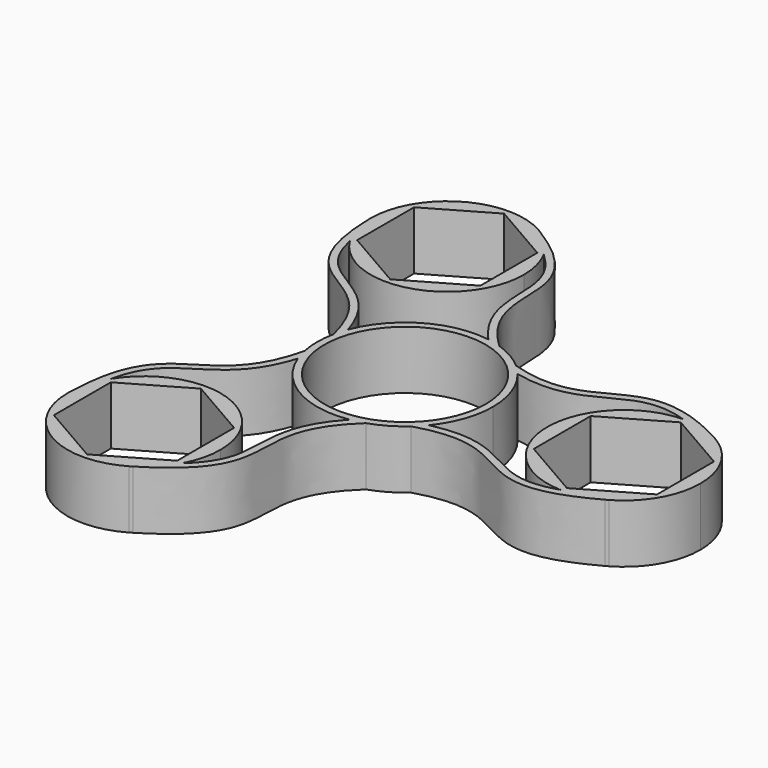
from build123d import *

# Parameters (mm, degrees)
F1_R     = 11.05
F2_DEPTH = 8


# Not quite as in the source:
# - the dataset's text gives a spline's control points without its knots; the knots are read off the source's solid


with BuildPart() as f2:
    # F1 (on Top) → F2 (new body)
    with BuildSketch(Plane.XY):
        with BuildLine():
            add(Edge.make_bspline(
                [(-23.9498664284, -20.4898704816), (-23.8093874058, -19.8426867285), (-23.468726692, -18.6366109287), (-22.828701594, -17.1870085553), (-22.0677112404, -16.020381617), (-21.2122966171, -15.0814244691), (-20.2601756399, -14.2881589816), (-18.8658523772, -13.3343486428), (-16.9218620299, -12.1842349069), (-14.8947876528, -10.62274426), (-13.3989040624, -8.8483289097), (-12.2627989857, -7.0040651939), (-11.5948300671, -5.3682178456), (-11.2616482193, -4.2869312315)],
                knots=[0.1298047456, 0.1298047456, 0.1298047456, 0.1298047456, 0.1875, 0.25, 0.3125, 0.375, 0.4375, 0.5, 0.625, 0.75, 0.8125, 0.875, 0.9599937126, 0.9599937126, 0.9599937126, 0.9599937126], degree=3))
            ThreePointArc((-11.2616482193, -4.2869312315), (-11.5680523877, -3.3738203797), (-11.8005517613, -2.4391552079))
            add(Edge.make_bspline(
                [(-25.4913456153, -25.5545377836), (-25.0594663371, -8.3982224046), (-14.9740294657, -16.111652051), (-11.8005517613, -2.4391552079)],
                knots=[0.221092115, 0.221092115, 0.221092115, 0.221092115, 27.237513428, 27.237513428, 27.237513428, 27.237513428], degree=3))
            ThreePointArc((-25.4913456153, -25.5545377836), (-25.0450433126, -22.923458588), (-23.9498664284, -20.4898704816))
        make_face()
        with BuildLine():
            add(Edge.make_bspline(
                [(3.7879055068, -11.4391552079), (-6.4660852403, -21.0237159398), (5.2566592195, -25.9012456555), (-9.3852060949, -34.8534217713)],
                knots=[0, 0, 0, 0, 27.016421313, 27.016421313, 27.016421313, 27.016421313], degree=3))
            ThreePointArc((3.7879055068, -11.4391552079), (2.8622120372, -11.70513743), (1.9182327589, -11.8963390622))
            add(Edge.make_bspline(
                [(1.9182327589, -11.8963390622), (1.1484020062, -12.7255263135), (0.0657011052, -14.12192804), (-0.9634255856, -16.0279557557), (-1.7521725606, -18.2106366213), (-2.0909259401, -20.7468798507), (-2.114958479, -23.0054817441), (-2.2438208314, -24.6899062801), (-2.454748407, -25.9110999776), (-2.8402018384, -27.1213893461), (-3.4700352269, -28.3637397934), (-4.4054151587, -29.6428189741), (-5.2795770833, -30.5408777063), (-5.7698151431, -30.9861279851)],
                knots=[0.0400062874, 0.0400062874, 0.0400062874, 0.0400062874, 0.125, 0.1875, 0.25, 0.375, 0.5, 0.5625, 0.625, 0.6875, 0.75, 0.8125, 0.8701952544, 0.8701952544, 0.8701952544, 0.8701952544], degree=3))
            ThreePointArc((-5.7698151431, -30.9861279851), (-7.3297758235, -33.1513730416), (-9.3852060949, -34.8534217713))
        make_face()
        with BuildLine():
            ThreePointArc((9.3434154605, 7.6094078307), (8.7058403505, 8.3313170502), (8.0126462545, 9))
            ThreePointArc((8.0126462545, 9), (6.025, 10.4356061156), (3.7879055068, 11.4391552079))
            ThreePointArc((3.7879055068, 11.4391552079), (2.8622120372, 11.70513743), (1.9182327589, 11.8963390622))
            ThreePointArc((1.9182327589, 11.8963390622), (-6.025, 10.4356061156), (-11.2616482193, 4.2869312315))
            ThreePointArc((-11.2616482193, 4.2869312315), (-11.5680523877, 3.3738203797), (-11.8005517613, 2.4391552079))
            ThreePointArc((-11.8005517613, 2.4391552079), (-12.05, 0), (-11.8005517613, -2.4391552079))
            ThreePointArc((-11.8005517613, -2.4391552079), (-11.5680523877, -3.3738203797), (-11.2616482193, -4.2869312315))
            ThreePointArc((-11.2616482193, -4.2869312315), (-6.025, -10.4356061156), (1.9182327589, -11.8963390622))
            ThreePointArc((1.9182327589, -11.8963390622), (2.8622120372, -11.70513743), (3.7879055068, -11.4391552079))
            ThreePointArc((3.7879055068, -11.4391552079), (6.025, -10.4356061156), (8.0126462545, -9))
            ThreePointArc((8.0126462545, -9), (8.7058403505, -8.3313170502), (9.3434154605, -7.6094078307))
            ThreePointArc((9.3434154605, -7.6094078307), (11.3532078352, -4.0382139432), (12.05, 0))
            ThreePointArc((12.05, 0), (11.3532078352, 4.0382139432), (9.3434154605, 7.6094078307))
        make_face()
        Circle(F1_R, mode=Mode.SUBTRACT)
        with BuildLine():
            add(Edge.make_bspline(
                [(-9.3852060949, -34.8534217713), (-9.5050295509, -34.9266829753), (-9.6266186878, -35.0002170649), (-9.75, -35.0740288533)],
                knots=[27.016421313, 27.016421313, 27.016421313, 27.016421313, 27.237513428, 27.237513428, 27.237513428, 27.237513428], degree=3))
            ThreePointArc((-9.3852060949, -34.8534217713), (-7.3297758235, -33.1513730416), (-5.7698151431, -30.9861279851))
            ThreePointArc((-5.7698151431, -30.9861279851), (-4.8224035009, -28.5627244489), (-4.5, -25.9807621135))
            ThreePointArc((-4.5, -25.9807621135), (-12.1472467245, -15.8757238281), (-23.9498664284, -20.4898704816))
            ThreePointArc((-23.9498664284, -20.4898704816), (-25.0450433126, -22.923458588), (-25.4913456153, -25.5545377836))
            add(Edge.make_bspline(
                [(-25.5, -25.9807621135), (-25.4977677723, -25.8370048686), (-25.4948799511, -25.6949385424), (-25.4913456153, -25.5545377836)],
                knots=[0, 0, 0, 0, 0.221092115, 0.221092115, 0.221092115, 0.221092115], degree=3))
            ThreePointArc((-25.5, -25.9807621135), (-20.25, -35.0740288533), (-9.75, -35.0740288533))
        make_face()
        Polygon((-23.45, -21.1021523389), (-15, -16.2235425642), (-6.55, -21.1021523389), (-6.55, -30.8593718882), (-15, -35.7379816628), (-23.45, -30.8593718882), align=None, mode=Mode.SUBTRACT)
        with BuildLine():
            ThreePointArc((35.25, -9.0932667397), (39.0932667397, -5.25), (40.5, 0))
            ThreePointArc((40.5, 0), (39.0932667397, 5.25), (35.25, 9.0932667397))
            add(Edge.make_bspline(
                [(34.8765517102, 9.2988839877), (34.9999095019, 9.2317444329), (35.1243864601, 9.1632121963), (35.25, 9.0932667397)],
                knots=[27.016421313, 27.016421313, 27.016421313, 27.016421313, 27.237513428, 27.237513428, 27.237513428, 27.237513428], degree=3))
            ThreePointArc((34.8765517102, 9.2988839877), (32.3748191361, 10.2279144536), (29.7196815716, 10.4962575034))
            ThreePointArc((29.7196815716, 10.4962575034), (19.5, 0), (29.7196815716, -10.4962575034))
            ThreePointArc((29.7196815716, -10.4962575034), (32.3748191361, -10.2279144536), (34.8765517102, -9.2988839877))
            add(Edge.make_bspline(
                [(34.8765517102, -9.2988839877), (34.9999095019, -9.2317444329), (35.1243864601, -9.1632121963), (35.25, -9.0932667397)],
                knots=[27.016421313, 27.016421313, 27.016421313, 27.016421313, 27.237513428, 27.237513428, 27.237513428, 27.237513428], degree=3))
        make_face()
        Polygon((21.55, 4.8786097747), (30, 9.7572195493), (38.45, 4.8786097747), (38.45, -4.8786097747), (30, -9.7572195493), (21.55, -4.8786097747), align=None, mode=Mode.SUBTRACT)
        with BuildLine():
            add(Edge.make_bspline(
                [(8.0126462545, -9), (21.440114706, -4.9120638887), (19.8028071176, -17.5030232509), (34.8765517102, -9.2988839877)],
                knots=[0, 0, 0, 0, 27.016421313, 27.016421313, 27.016421313, 27.016421313], degree=3))
            ThreePointArc((34.8765517102, -9.2988839877), (32.3748191361, -10.2279144536), (29.7196815716, -10.4962575034))
            add(Edge.make_bspline(
                [(9.3434154605, -7.6094078307), (10.4464280609, -7.3573084679), (12.1970978805, -7.1178628462), (14.362329648, -7.1796268461), (16.6469602135, -7.5878923613), (19.01278797, -8.5626449438), (20.9808108562, -9.6711331013), (22.5039964713, -10.4017472985), (23.6670450241, -10.8296755084), (24.9079130788, -11.1010077291), (26.2987368209, -11.1767312382), (27.8741418507, -11.0062080454), (29.0889644891, -10.6981909778), (29.7196815716, -10.4962575034)],
                knots=[0.0400062874, 0.0400062874, 0.0400062874, 0.0400062874, 0.125, 0.1875, 0.25, 0.375, 0.5, 0.5625, 0.625, 0.6875, 0.75, 0.8125, 0.8701952544, 0.8701952544, 0.8701952544, 0.8701952544], degree=3))
            ThreePointArc((9.3434154605, -7.6094078307), (8.7058403505, -8.3313170502), (8.0126462545, -9))
        make_face()
        with BuildLine():
            ThreePointArc((29.7196815716, 10.4962575034), (32.3748191361, 10.2279144536), (34.8765517102, 9.2988839877))
            add(Edge.make_bspline(
                [(8.0126462545, 9), (21.440114706, 4.9120638887), (19.8028071176, 17.5030232509), (34.8765517102, 9.2988839877)],
                knots=[0, 0, 0, 0, 27.016421313, 27.016421313, 27.016421313, 27.016421313], degree=3))
            ThreePointArc((8.0126462545, 9), (8.7058403505, 8.3313170502), (9.3434154605, 7.6094078307))
            add(Edge.make_bspline(
                [(9.3434154605, 7.6094078307), (10.4464280609, 7.3573084679), (12.1970978805, 7.1178628462), (14.362329648, 7.1796268461), (16.6469602135, 7.5878923613), (19.01278797, 8.5626449438), (20.9808108562, 9.6711331013), (22.5039964713, 10.4017472985), (23.6670450241, 10.8296755084), (24.9079130788, 11.1010077291), (26.2987368209, 11.1767312382), (27.8741418507, 11.0062080454), (29.0889644891, 10.6981909778), (29.7196815716, 10.4962575034)],
                knots=[0.0400062874, 0.0400062874, 0.0400062874, 0.0400062874, 0.125, 0.1875, 0.25, 0.375, 0.5, 0.5625, 0.625, 0.6875, 0.75, 0.8125, 0.8701952544, 0.8701952544, 0.8701952544, 0.8701952544], degree=3))
        make_face()
        with BuildLine():
            ThreePointArc((-11.8005517613, 2.4391552079), (-11.5680523877, 3.3738203797), (-11.2616482193, 4.2869312315))
            add(Edge.make_bspline(
                [(-23.9498664284, 20.4898704816), (-23.8093874058, 19.8426867285), (-23.468726692, 18.6366109287), (-22.828701594, 17.1870085553), (-22.0677112404, 16.020381617), (-21.2122966171, 15.0814244691), (-20.2601756399, 14.2881589816), (-18.8658523772, 13.3343486428), (-16.9218620299, 12.1842349069), (-14.8947876528, 10.62274426), (-13.3989040624, 8.8483289097), (-12.2627989857, 7.0040651939), (-11.5948300671, 5.3682178456), (-11.2616482193, 4.2869312315)],
                knots=[0.1298047456, 0.1298047456, 0.1298047456, 0.1298047456, 0.1875, 0.25, 0.3125, 0.375, 0.4375, 0.5, 0.625, 0.75, 0.8125, 0.875, 0.9599937126, 0.9599937126, 0.9599937126, 0.9599937126], degree=3))
            ThreePointArc((-23.9498664284, 20.4898704816), (-25.0450433126, 22.923458588), (-25.4913456153, 25.5545377836))
            add(Edge.make_bspline(
                [(-25.4913456153, 25.5545377836), (-25.0594663371, 8.3982224046), (-14.9740294657, 16.111652051), (-11.8005517613, 2.4391552079)],
                knots=[0.221092115, 0.221092115, 0.221092115, 0.221092115, 27.237513428, 27.237513428, 27.237513428, 27.237513428], degree=3))
        make_face()
        with BuildLine():
            ThreePointArc((-5.7698151431, 30.9861279851), (-7.3297758235, 33.1513730416), (-9.3852060949, 34.8534217713))
            add(Edge.make_bspline(
                [(-9.75, 35.0740288533), (-9.6266186878, 35.0002170649), (-9.5050295509, 34.9266829753), (-9.3852060949, 34.8534217713)],
                knots=[0, 0, 0, 0, 0.221092115, 0.221092115, 0.221092115, 0.221092115], degree=3))
            ThreePointArc((-9.75, 35.0740288533), (-20.25, 35.0740288533), (-25.5, 25.9807621135))
            add(Edge.make_bspline(
                [(-25.5, 25.9807621135), (-25.4977677723, 25.8370048686), (-25.4948799511, 25.6949385424), (-25.4913456153, 25.5545377836)],
                knots=[0, 0, 0, 0, 0.221092115, 0.221092115, 0.221092115, 0.221092115], degree=3))
            ThreePointArc((-25.4913456153, 25.5545377836), (-25.0450433126, 22.923458588), (-23.9498664284, 20.4898704816))
            ThreePointArc((-23.9498664284, 20.4898704816), (-12.1472467245, 15.8757238281), (-4.5, 25.9807621135))
            ThreePointArc((-4.5, 25.9807621135), (-4.8224035009, 28.5627244489), (-5.7698151431, 30.9861279851))
        make_face()
        Polygon((-6.55, 30.8593718882), (-6.55, 21.1021523389), (-15, 16.2235425642), (-23.45, 21.1021523389), (-23.45, 30.8593718882), (-15, 35.7379816628), align=None, mode=Mode.SUBTRACT)
        with BuildLine():
            ThreePointArc((1.9182327589, 11.8963390622), (2.8622120372, 11.70513743), (3.7879055068, 11.4391552079))
            add(Edge.make_bspline(
                [(-9.3852060949, 34.8534217713), (5.2566592195, 25.9012456555), (-6.4660852403, 21.0237159398), (3.7879055068, 11.4391552079)],
                knots=[0.221092115, 0.221092115, 0.221092115, 0.221092115, 27.237513428, 27.237513428, 27.237513428, 27.237513428], degree=3))
            ThreePointArc((-9.3852060949, 34.8534217713), (-7.3297758235, 33.1513730416), (-5.7698151431, 30.9861279851))
            add(Edge.make_bspline(
                [(-5.7698151431, 30.9861279851), (-5.2795770833, 30.5408777063), (-4.4054151587, 29.6428189741), (-3.4700352269, 28.3637397934), (-2.8402018384, 27.1213893461), (-2.454748407, 25.9110999776), (-2.2438208314, 24.6899062801), (-2.114958479, 23.0054817441), (-2.0909259401, 20.7468798507), (-1.7521725606, 18.2106366213), (-0.9634255856, 16.0279557557), (0.0657011052, 14.12192804), (1.1484020062, 12.7255263135), (1.9182327589, 11.8963390622)],
                knots=[0.1298047456, 0.1298047456, 0.1298047456, 0.1298047456, 0.1875, 0.25, 0.3125, 0.375, 0.4375, 0.5, 0.625, 0.75, 0.8125, 0.875, 0.9599937126, 0.9599937126, 0.9599937126, 0.9599937126], degree=3))
        make_face()
    extrude(amount=F2_DEPTH)


solid = f2.part
